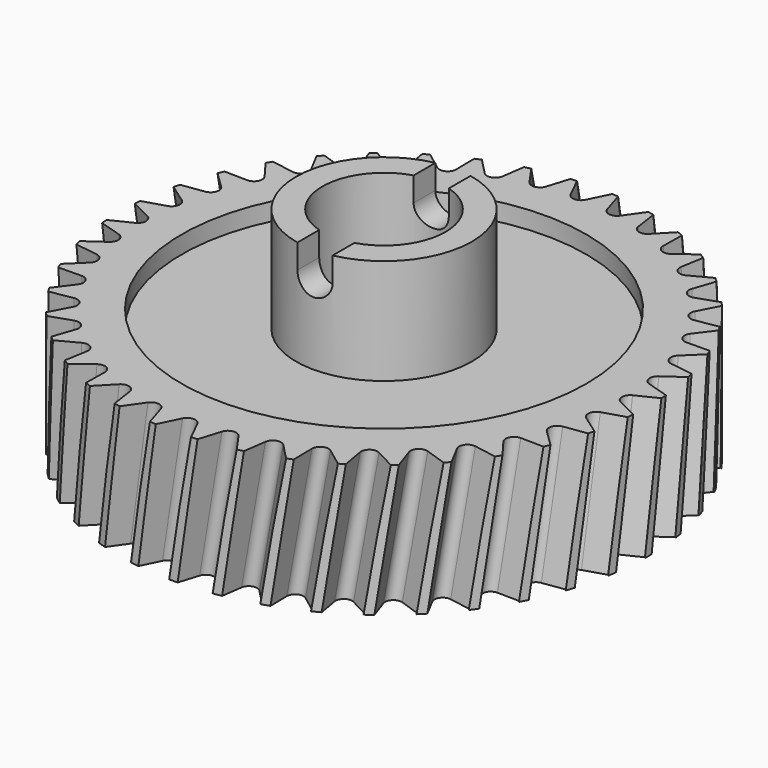
from build123d import *

# Parameters (mm, degrees)
F0_R             = 30
F1_DEPTH         = 15
F2_R             = 23
F3_DEPTH         = 2
F4_R             = 10
F5_DEPTH         = 12
F6_R             = 7
F7_DEPTH         = 45.4
F9_DEPTH         = 12.5
F12_COPIES_COUNT = 40


# Not quite as in the source:
# - a pattern or mirror of a feature is missing from the dataset's text; its kind, count and spacing are read off the source's solid


with BuildPart() as f1:
    # F0 (on Top) → F1 (new body)
    with BuildSketch(Plane.XY):
        Circle(F0_R)
    extrude(amount=F1_DEPTH)

    # F2 (on face) → F3 (cut)
    with BuildSketch(Plane.XY.offset(15)):
        Circle(F2_R)
    extrude(amount=-F3_DEPTH, mode=Mode.SUBTRACT)

    # F4 (on face) → F5 (join)
    with BuildSketch(Plane.XY.offset(13)):
        Circle(F4_R)
    extrude(amount=F5_DEPTH)

    # F6 (on face) → F7 (cut)
    with BuildSketch(Plane.XY.offset(25)):
        Circle(F6_R)
    extrude(amount=-F7_DEPTH, mode=Mode.SUBTRACT)

    # F8 (on Front) → F9 (cut, symmetric)
    with BuildSketch(Plane.XZ):
        with BuildLine():
            Line((2, 22.2432126286), (2, 26.2432126286))
            Line((2, 26.2432126286), (-2, 26.2432126286))
            Line((-2, 26.2432126286), (-2, 22.2432126286))
            ThreePointArc((-2, 22.2432126286), (0, 20.2432126286), (2, 22.2432126286))
        make_face()
    extrude(amount=F9_DEPTH, both=True, mode=Mode.SUBTRACT)

    # F12: sweep along a path in F11
    with BuildLine(Plane.XZ) as f12_path:
        Line((0, -1.2824153311), (-2.5731360074, 15.7175846689))
    # F10 (on face) → F12 (sweep, cut)
    with BuildSketch(Plane.XY.offset(15)):
        with BuildLine():
            Line((-2, 29.9332590942), (-0.8464378818, 27.5843157777))
            ThreePointArc((-0.8464378818, 27.5843157777), (0, 27.0569992257), (0.8464378818, 27.5843157777))
            Line((0.8464378818, 27.5843157777), (2, 29.9332590942))
            ThreePointArc((2, 29.9332590942), (0, 30), (-2, 29.9332590942))
        make_face()
        with BuildLine():
            ThreePointArc((2, 29.9332590942), (0, 30.3449676591), (-2, 29.9332590942))
            ThreePointArc((-2, 29.9332590942), (0, 30), (2, 29.9332590942))
        make_face()
    f12 = sweep(path=f12_path.line, mode=Mode.SUBTRACT)

    # F12_copies: F12 ×40 about axis
    f12_copies_axis = Axis((0, 0, 0), (0, 0, 1))
    for i in range(1, F12_COPIES_COUNT):
        add(f12.rotate(f12_copies_axis, i * 360 / F12_COPIES_COUNT), mode=Mode.SUBTRACT)


solid = f1.part
